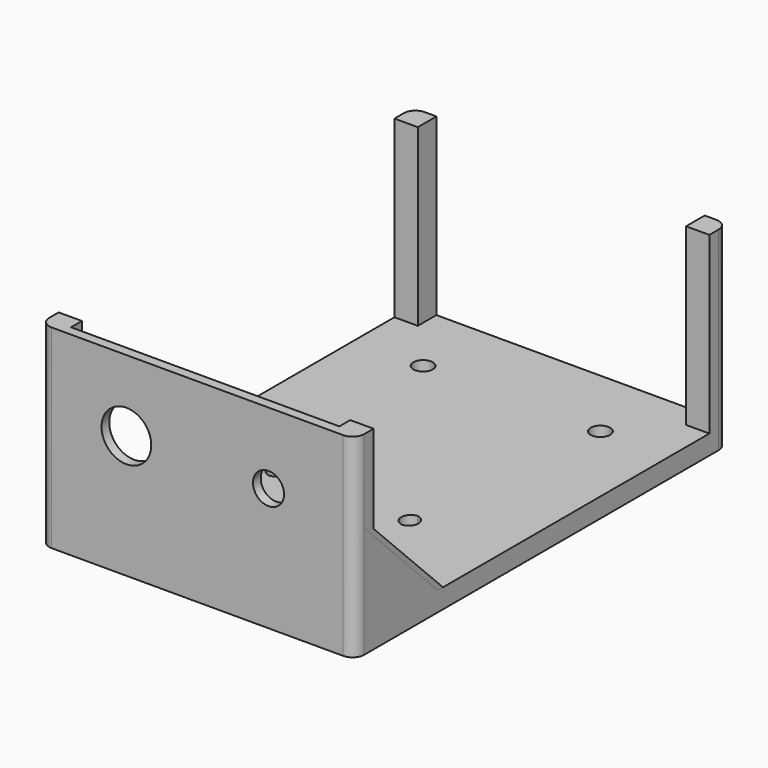
from build123d import *

# Parameters (mm, degrees)
F0_W         = 88.9
F0_H         = 63.5
F1_DEPTH     = 3.174
F2_W         = 88.9
F2_H         = 149.226
F3_DEPTH     = 6.35
F4_W         = 34.926
F4_H         = 33.8644637015
F5_DEPTH     = 6.35
F6_W         = 37.0404637015
F6_H         = 33.8644637015
F7_DEPTH     = 6.35
F8_T4_DEPTH  = 6.35
F9_T4_DEPTH  = 6.35
F10_R        = 8
F11_DEPTH    = 152.401
F10_R_2      = 5
F12_DEPTH    = 25.4
F13_R        = 3.175
F14_DEPTH    = 25.4
F15_DEPTH    = 7
F16_DEPTH    = 7
F17_DEPTH    = 7
F18_DEPTH    = 7
F19_W        = 7.62
F19_H        = 7.62
F20_DEPTH    = 63.5
F21_W        = 7.62
F21_H        = 63.5
F22_DEPTH    = 7.62
F24_T1_DEPTH = 82.55
F25_T1_DEPTH = 82.55
F26_R        = 3.81
F28_R        = 3.175
F29_DEPTH    = 25.4
F30_R        = 8.128
F31_DEPTH    = 25.4
F32_R        = 5.08
F33_DEPTH    = 25.4


# Not quite as in the source:
# - a fillet or chamfer that OpenCascade refuses, or shapes differently, is made with other operations: its cross-section is extruded or revolved along the edge and cut away or added
# - two fillets or chamfers of one size are made in one step


with BuildPart() as f1:
    # F0 (on Front) → F1 (new body)
    with BuildSketch(Plane.XZ):
        with Locations((8.606e-07, -8.4644637015)):
            Rectangle(F0_W, F0_H)
    extrude(amount=-F1_DEPTH)

    # F2 (on face) → F3 (join)
    with BuildSketch(Plane(origin=(0, 0, -40.2144637015), x_dir=(1, 0, 0), z_dir=(0, 0, -1))):
        with Locations((8.606e-07, -77.787)):
            Rectangle(F2_W, F2_H)
    extrude(amount=-F3_DEPTH)

    # F4 (on face) → F5 (join)
    with BuildSketch(Plane.YZ.offset(44.4500008606)):
        with Locations((20.637, -16.9322318508)):
            Rectangle(F4_W, F4_H)
    extrude(amount=-F5_DEPTH)

    # F6 (on face) → F7 (join)
    with BuildSketch(Plane(origin=(-44.4499991394, 0, 0), x_dir=(0, -1, 0), z_dir=(-1, 0, 0))):
        with Locations((-21.6942318508, -16.9322318508)):
            Rectangle(F6_W, F6_H)
    extrude(amount=-F7_DEPTH)

    # F8: chamfer of 38.1 on 1 edges, made by hand


with BuildPart() as f8_tool2:
    # F8_s3 → F8_t4 (new body)
    with BuildSketch(Plane.YZ.offset(-44.4499991394)):
        with BuildLine():
            Line((1.036832967, 1.0776307345), (41.292094436, -39.1776307345))
            Line((41.292094436, -39.1776307345), (42.054094436, -39.1776307345))
            ThreePointArc((42.054094436, -39.1776307345), (40.9764637015, -19.5888153673), (40.9764637015, 0))
            Line((40.9764637015, 0), (40.2144637015, 0.762))
            ThreePointArc((40.2144637015, 0.762), (20.6256483342, 0.762), (1.036832967, 1.8396307345))
            Line((1.036832967, 1.8396307345), (1.036832967, 1.0776307345))
        make_face()
    extrude(amount=F8_T4_DEPTH)

    split(bisect_by=Plane.XZ.offset(-3.174), keep=Keep.BOTTOM)

    split(bisect_by=Plane.XY.offset(-33.8644637015), keep=Keep.TOP)


with BuildPart() as f1_1:
    add(f1.part)

    # F8_t1: cut F8_tool2
    add(f8_tool2.part, mode=Mode.SUBTRACT)

    # F9: chamfer of 38.1 on 1 edges, made by hand


with BuildPart() as f9_tool2:
    # F9_s3 → F9_t4 (new body)
    with BuildSketch(Plane.YZ.offset(44.4500008606)):
        with BuildLine():
            Line((-1.0776307345, 1.0776307345), (39.1776307345, -39.1776307345))
            Line((39.1776307345, -39.1776307345), (39.9396307345, -39.1776307345))
            ThreePointArc((39.9396307345, -39.1776307345), (38.862, -19.5888153673), (38.862, 0))
            Line((38.862, 0), (38.1, 0.762))
            ThreePointArc((38.1, 0.762), (18.5111846327, 0.762), (-1.0776307345, 1.8396307345))
            Line((-1.0776307345, 1.8396307345), (-1.0776307345, 1.0776307345))
        make_face()
    extrude(amount=-F9_T4_DEPTH)

    split(bisect_by=Plane.XZ.offset(-3.174), keep=Keep.BOTTOM)

    split(bisect_by=Plane.XY.offset(-33.8644637015), keep=Keep.TOP)


with BuildPart() as f1_2:
    add(f1_1.part)

    # F9_t1: cut F9_tool2
    add(f9_tool2.part, mode=Mode.SUBTRACT)

    # F10 (on face) → F11 (cut, through all)
    with BuildSketch(Plane.XZ):
        with Locations((-23.4761538258, 0)):
            Circle(F10_R)
    extrude(amount=-F11_DEPTH, mode=Mode.SUBTRACT)

    # F10 (on face) → F12 (cut)
    with BuildSketch(Plane.XZ):
        with Locations((-23.4761538258, 0)):
            Circle(F10_R)
        with Locations((23.2181741801, 0)):
            Circle(F10_R_2)
    extrude(amount=-F12_DEPTH, mode=Mode.SUBTRACT)

    # F13 (on face) → F14 (cut)
    with BuildSketch(Plane.XY.offset(-33.8644637015)):
        with Locations((0, 18.4923222025)):
            Circle(F13_R)
        with Locations((-22.079911083, 59.5920197666)):
            Circle(F13_R)
        with Locations((21.367656067, 59.5920197666)):
            Circle(F13_R)
    extrude(amount=-F14_DEPTH, mode=Mode.SUBTRACT)

    # F15 (add): a face of the model
    f15_faces = [f1_2.faces().sort_by_distance(p)[0] for p in [
        (44.4500008606, 76.2, -38.5634637015),
    ]]
    extrude(f15_faces, amount=F15_DEPTH)

    # F16 (add): a face of the model
    f16_faces = [f1_2.faces().sort_by_distance(p)[0] for p in [
        (-44.4499991394, 1.651, -8.4644637015),
    ]]
    extrude(f16_faces, amount=F16_DEPTH)

    # F17 (cut): a face of the model
    f17_faces = [f1_2.faces().sort_by_distance(p)[0] for p in [
        (38.1000008606, 13.4041545672, -23.6343091343),
    ]]
    extrude(f17_faces, amount=-F17_DEPTH, mode=Mode.SUBTRACT)

    # F18 (cut): a face of the model
    f18_faces = [f1_2.faces().sort_by_distance(p)[0] for p in [
        (-38.0999991394, 14.108975801, -22.9294879005),
    ]]
    extrude(f18_faces, amount=-F18_DEPTH, mode=Mode.SUBTRACT)

    # F19 (on face) → F20 (join)
    with BuildSketch(Plane(origin=(0, 0, -40.2144637015), x_dir=(1, 0, 0), z_dir=(0, 0, -1))):
        with Locations((47.6400008606, -148.59)):
            Rectangle(F19_W, F19_H)
    extrude(amount=-F20_DEPTH)

    # F21 (on face) → F22 (join)
    with BuildSketch(Plane.XZ):
        with Locations((-47.6399991394, -8.4644637015)):
            Rectangle(F21_W, F21_H)
    extrude(amount=-F22_DEPTH)

    # F23: F1 across plane


with BuildPart() as f1_3:
    add(f1_2.part)
    add(f1_2.part.mirror(Plane.YZ))

    # F24: fillet of radius 3.81 on 1 edges, made by hand

    # F24_s2 → F24_t1 (cut)
    with BuildSketch(Plane.XY.offset(-49.7394637015)):
        with BuildLine():
            ThreePointArc((47.6400008606, 0), (50.3340776969, 1.1159231637), (51.4500008606, 3.81))
            Line((51.4500008606, 3.81), (51.4500008606, 0))
            Line((51.4500008606, 0), (47.6400008606, 0))
        make_face()
    extrude(amount=F24_T1_DEPTH, mode=Mode.SUBTRACT)

    # F25: fillet of radius 3.81 on 1 edges, made by hand

    # F25_s2 → F25_t1 (cut)
    with BuildSketch(Plane.XY.offset(-49.7394637015)):
        with BuildLine():
            ThreePointArc((-51.4500008606, 3.81), (-50.3340776969, 1.1159231637), (-47.6400008606, 0))
            Line((-47.6400008606, 0), (-51.4500008606, 0))
            Line((-51.4500008606, 0), (-51.4500008606, 3.81))
        make_face()
    extrude(amount=F25_T1_DEPTH, mode=Mode.SUBTRACT)

    # F26
    f26_edges = [f1_3.edges().sort_by_distance(p)[0] for p in [
        (51.450001, 152.4, -8.464464),
        (-51.450001, 152.4, -8.464464),
    ]]
    fillet(f26_edges, radius=F26_R)

    # F28 (on face) → F29 (cut)
    with BuildSketch(Plane.XY.offset(-33.8644637015)):
        with Locations((28.9712660015, 128.3781081438)):
            Circle(F28_R)
        with Locations((-28.9712660015, 128.3781081438)):
            Circle(F28_R)
    extrude(amount=-F29_DEPTH, mode=Mode.SUBTRACT)

    # F30 (on face) → F31 (cut)
    with BuildSketch(Plane.XZ):
        with Locations((-23.2181741801, 0)):
            Circle(F30_R)
    extrude(amount=-F31_DEPTH, mode=Mode.SUBTRACT)

    # F32 (on face) → F33 (cut)
    with BuildSketch(Plane.XZ):
        with Locations((23.2181741801, 0)):
            Circle(F32_R)
    extrude(amount=-F33_DEPTH, mode=Mode.SUBTRACT)


solid = f1_3.part
